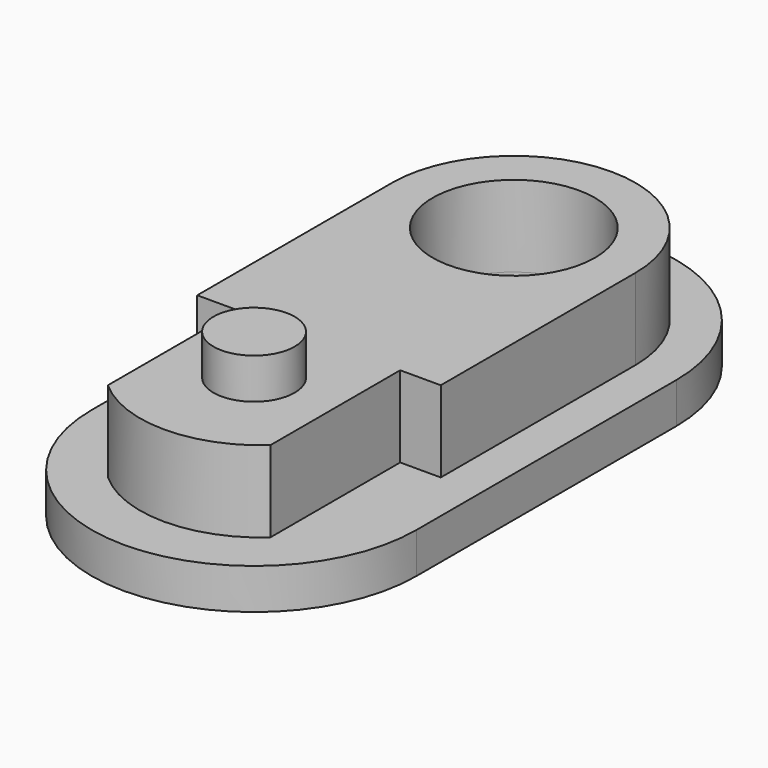
from build123d import *

# Parameters (mm, degrees)
F1_DEPTH = 12.7
F2_R     = 6.35
F3_DEPTH = 6.35
F5_DEPTH = 6.35
F6_DEPTH = 6.35
F7_R     = 12.7
F8_DEPTH = 19.051


# Not quite as in the source:
# - ends of sketch curves that miss each other by under 0.0002 mm in the source are joined


with BuildPart() as f1:
    # F0 (on Top) → F1 (new body)
    with BuildSketch(Plane.XY):
        with BuildLine():
            Line((19.05, -12.7), (19.05, 25.4))
            ThreePointArc((19.05, 25.4), (-0.0047443873, 44.4452550218), (-19.0499994092, 25.3905112253))
            Line((-19.0499994092, 25.3905112253), (-19.05, -12.7))
            Line((-19.05, -12.7), (-12.7, -12.7))
            Line((-12.7, -12.7), (-12.7, -38.1))
            ThreePointArc((-12.7, -38.1), (0, -42.9509683429), (12.7, -38.1))
            Line((12.7, -38.1), (12.7, -12.7))
            Line((12.7, -12.7), (19.05, -12.7))
        make_face()
    extrude(amount=-F1_DEPTH)

    # F2 (on face) → F3 (join)
    with BuildSketch(Plane.XY):
        with Locations((0, -25.4)):
            Circle(F2_R)
    extrude(amount=F3_DEPTH)


with BuildPart() as f5:
    # F4 (on face) → F5 (new body)
    with BuildSketch(Plane(origin=(0, 0, -12.7), x_dir=(1, 0, 0), z_dir=(0, 0, -1))):
        with BuildLine():
            Line((25.4189755796, -25.3984153871), (25.4063238802, 25.4015830374))
            ThreePointArc((25.4063238802, 25.4015830374), (-0.0063274248, 50.8015794928), (-25.4063238802, 25.3889281877))
            Line((-25.4063238802, 25.3889281877), (-25.3936721808, -25.4110702368))
            ThreePointArc((-25.3936721808, -25.4110702368), (0.0189791242, -50.8110666922), (25.4189755796, -25.3984153871))
        make_face()
        with BuildLine():
            Line((12.7, 38.1), (12.7, 25.3952556126))
            Line((12.7, 25.3952556126), (12.7, 12.7))
            Line((12.7, 12.7), (19.05, 12.7))
            Line((19.05, 12.7), (19.05, -25.4))
            ThreePointArc((19.05, -25.4), (-0.0047440919, -44.4452550219), (-19.0499994092, -25.3905112253))
            Line((-19.0499994092, -25.3905112253), (-19.05, 12.7))
            Line((-19.05, 12.7), (-12.7, 12.7))
            Line((-12.7, 12.7), (-12.7, 25.3952556126))
            Line((-12.7, 25.3952556126), (-12.7, 38.1))
            ThreePointArc((-12.7, 38.1), (-6.7996767952, 41.696105192), (-0.0047443873, 42.9509677521))
            ThreePointArc((-0.0047443873, 42.9509677521), (6.7952447197, 41.6977980942), (12.7, 38.1))
        make_face(mode=Mode.SUBTRACT)
    extrude(amount=F5_DEPTH)


with BuildPart() as f6:
    # F6 (new): a face of the model
    f6_faces = [f1.part.faces().sort_by_distance(p)[0] for p in [
        (1.391e-07, 3.0992224533, -12.7),
    ]]
    extrude(f6_faces, amount=F6_DEPTH)


with BuildPart() as f8_tool:
    # F7 (on face) → F8 (new body, through all)
    with BuildSketch(Plane.XY):
        with Locations((2.954e-07, 25.3952556127)):
            Circle(F7_R)
    extrude(amount=-F8_DEPTH)


with BuildPart() as f1_1:
    add(f1.part)

    # F8: cut by f8_tool
    add(f8_tool.part, mode=Mode.SUBTRACT)


with BuildPart() as f6_1:
    add(f6.part)

    # F8: cut by f8_tool
    add(f8_tool.part, mode=Mode.SUBTRACT)


solid = Compound([f5.part, f1_1.part, f6_1.part])
